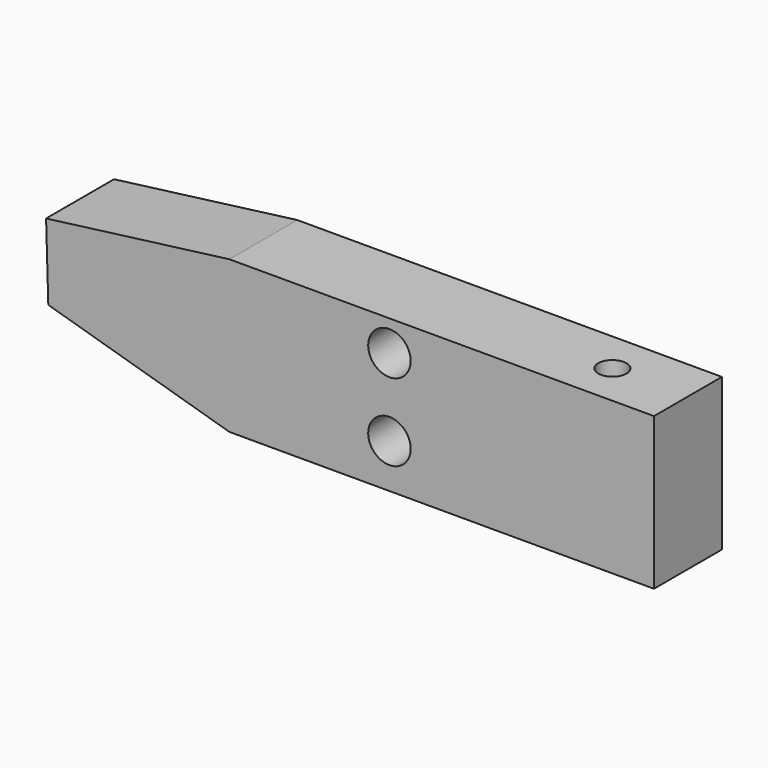
from build123d import *

# Parameters (mm, degrees)
F0_W     = 25
F0_H     = 17.9
F1_DEPTH = 10
F3_D     = 5
F4_W     = 10
F4_H     = 17.9
F5_DEPTH = 25
F6_R     = 1.66
F7_DEPTH = 25


# Not quite as in the source:
# - a feature names something its author has since deleted; it is built from what else it names


with BuildPart() as f1:
    # F0 (on Front) → F1 (new body)
    with BuildSketch(Plane.XZ):
        Polygon((-11.5858212113, -12.1098860052), (-11.5858212113, 5.7901139948), (-33.1716425717, 3.0010114424), (-32.9104475677, -5.8795856312), align=None)
        with Locations((0.9141787887, -3.1598860052)):
            Rectangle(F0_W, F0_H)
    extrude(amount=F1_DEPTH)

    # F3 (through all)
    with Locations(Plane.XZ.offset(10)):
        with Locations((7.2585181333, 2.1878613625), (7.2585181333, -6.9218412973)):
            Hole(F3_D / 2)

    # F4 (on face) → F5 (join)
    with BuildSketch(Plane.YZ.offset(13.4141787887)):
        with Locations((-5, -3.1598860052)):
            Rectangle(F4_W, F4_H)
    extrude(amount=F5_DEPTH)

    # F6 (on face) → F7 (cut)
    with BuildSketch(Plane.XY.offset(5.7901139948)):
        with Locations((29.4916108251, -4.9681207165)):
            Circle(F6_R)
    extrude(amount=-F7_DEPTH, mode=Mode.SUBTRACT)


solid = f1.part
